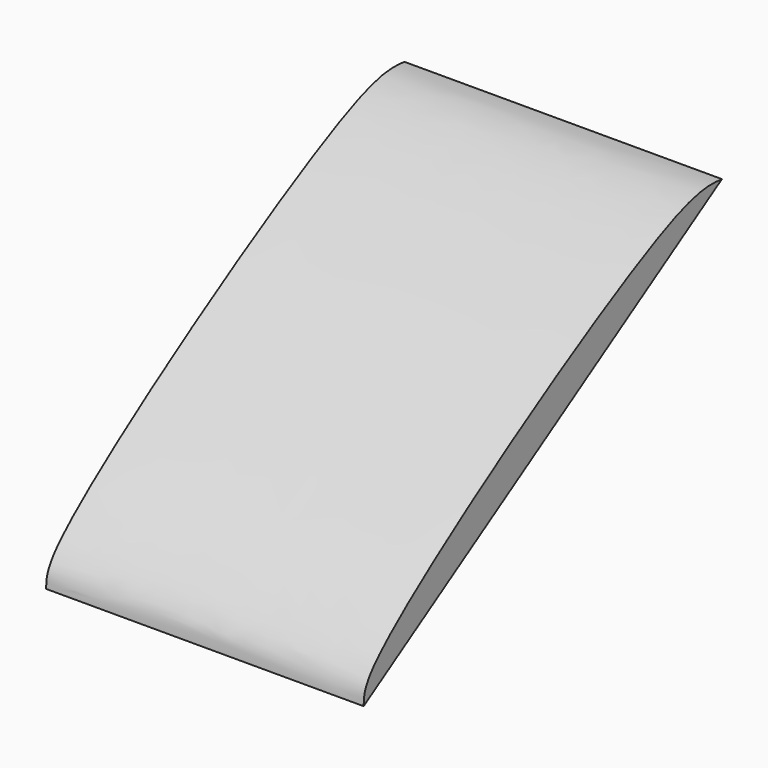
from build123d import *

# Parameters (mm, degrees)
F1_DEPTH  = 457.2
F2_W      = 63.5
F2_H      = 101.6
F3_DEPTH  = 50.8
F5_DEPTH  = 127
F7_DEPTH  = 6.35
F9_DEPTH  = 6.35
F11_DEPTH = 7.62
F12_W     = 19.05
F12_H     = 38.1
F13_DEPTH = 6.35
F14_W     = 9.525
F14_H     = 114.3
F15_DEPTH = 6.35
F17_DEPTH = 19.05
F19_DEPTH = 19.05
F21_DEPTH = 19.05
F23_DEPTH = 127


with BuildPart() as f1:
    # F0 (on Right) → F1 (new body)
    with BuildSketch(Plane.YZ):
        with BuildLine():
            Line((-644.8294241484, -406.0037115008), (0, 0))
            add(Edge.make_bspline(
                [(-644.8294241484, -406.0037115008), (-644.5583562129, -393.7520607079), (-643.3425508393, -338.8004381801), (-93.9791762847, 8.8024420181), (-20.2683336801, 1.8984081269), (0, 0)],
                knots=[0, 0, 0, 0, 0.1722048446, 0.7723804554, 1, 1, 1, 1], degree=3))
        make_face()
    extrude(amount=F1_DEPTH)

    # F2 (on face) → F3 (join)
    with BuildSketch(Plane(origin=(0, 0, 0), x_dir=(1, 0, 0), z_dir=(0, 0.5328132697, -0.8462328401))):
        with Locations((228.6, 381)):
            Rectangle(F2_W, F2_H)
    extrude(amount=F3_DEPTH)

    # F4 (on face) → F5 (cut)
    with BuildSketch(Plane(origin=(196.85, 0, 0), x_dir=(0, -1, 0), z_dir=(-1, 0, 0))):
        with BuildLine():
            Line((287.9840051675, -233.8501769674), (284.600640905, -239.223755502))
            Line((284.600640905, -239.223755502), (306.0949550433, -252.757212552))
            Line((306.0949550433, -252.757212552), (309.4783193058, -247.3836340174))
            Line((309.4783193058, -247.3836340174), (330.9726334441, -260.9170910675))
            ThreePointArc((330.9726334441, -260.9170910675), (317.4401312079, -210.9026606557), (266.4896910292, -220.3167199174))
            Line((266.4896910292, -220.3167199174), (287.9840051675, -233.8501769674))
        make_face()
    extrude(amount=-F5_DEPTH, mode=Mode.SUBTRACT)

    # F6 (on face) → F7 (join)
    with BuildSketch(Plane(origin=(196.85, 0, 0), x_dir=(0, -1, 0), z_dir=(-1, 0, 0))):
        with BuildLine():
            Line((252.3591696976, -218.9235699269), (284.600640905, -239.223755502))
            Line((284.600640905, -239.223755502), (287.9840051675, -233.8501769674))
            Line((287.9840051675, -233.8501769674), (266.4896910292, -220.3167199174))
            ThreePointArc((266.4896910292, -220.3167199174), (317.4401312079, -210.9026606557), (330.9726334441, -260.9170910675))
            Line((330.9726334441, -260.9170910675), (309.4783193058, -247.3836340174))
            Line((309.4783193058, -247.3836340174), (306.0949550433, -252.757212552))
            Line((306.0949550433, -252.757212552), (338.3364262507, -273.057398127))
            Line((338.3364262507, -273.057398127), (365.4033403508, -230.0687698505))
            Line((365.4033403508, -230.0687698505), (279.4260837976, -175.9349416504))
            Line((279.4260837976, -175.9349416504), (252.3591696976, -218.9235699269))
        make_face()
        with BuildLine():
            Line((287.9840051675, -233.8501769674), (284.600640905, -239.223755502))
            Line((284.600640905, -239.223755502), (306.0949550433, -252.757212552))
            Line((306.0949550433, -252.757212552), (309.4783193058, -247.3836340174))
            Line((309.4783193058, -247.3836340174), (330.9726334441, -260.9170910675))
            ThreePointArc((330.9726334441, -260.9170910675), (317.4401312079, -210.9026606557), (266.4896910292, -220.3167199174))
            Line((266.4896910292, -220.3167199174), (287.9840051675, -233.8501769674))
        make_face()
    extrude(amount=F7_DEPTH)

    # F8 (on face) → F9 (join)
    with BuildSketch(Plane.YZ.offset(260.35)):
        with BuildLine():
            Line((-338.3364262507, -273.057398127), (-306.0949550433, -252.757212552))
            Line((-306.0949550433, -252.757212552), (-309.4783193058, -247.3836340174))
            Line((-309.4783193058, -247.3836340174), (-330.9726334441, -260.9170910675))
            ThreePointArc((-330.9726334441, -260.9170910675), (-317.4401312079, -210.9026606557), (-266.4896910292, -220.3167199174))
            Line((-266.4896910292, -220.3167199174), (-287.9840051675, -233.8501769674))
            Line((-287.9840051675, -233.8501769674), (-284.600640905, -239.223755502))
            Line((-284.600640905, -239.223755502), (-252.3591696976, -218.9235699269))
            Line((-252.3591696976, -218.9235699269), (-279.4260837976, -175.9349416504))
            Line((-279.4260837976, -175.9349416504), (-365.4033403508, -230.0687698505))
            Line((-365.4033403508, -230.0687698505), (-338.3364262507, -273.057398127))
        make_face()
        with BuildLine():
            Line((-309.4783193058, -247.3836340174), (-306.0949550433, -252.757212552))
            Line((-306.0949550433, -252.757212552), (-284.600640905, -239.223755502))
            Line((-284.600640905, -239.223755502), (-287.9840051675, -233.8501769674))
            Line((-287.9840051675, -233.8501769674), (-266.4896910292, -220.3167199174))
            ThreePointArc((-266.4896910292, -220.3167199174), (-317.4401312079, -210.9026606557), (-330.9726334441, -260.9170910675))
            Line((-330.9726334441, -260.9170910675), (-309.4783193058, -247.3836340174))
        make_face()
    extrude(amount=F9_DEPTH)

    # F10 (on face) → F11 (cut)
    with BuildSketch(Plane(origin=(0, 27.0669141001, -42.9886282766), x_dir=(1, 0, 0), z_dir=(0, 0.5328132697, -0.8462328401))):
        with BuildLine():
            Line((260.35, 368.3), (196.85, 368.3))
            ThreePointArc((196.85, 368.3), (228.6, 364.3836558631), (260.35, 368.3))
        make_face()
        with BuildLine():
            ThreePointArc((260.35, 393.7), (228.6, 398.6686937584), (196.85, 393.7))
            Line((196.85, 393.7), (260.35, 393.7))
        make_face()
    extrude(amount=-F11_DEPTH, mode=Mode.SUBTRACT)

    # F12 (on face) → F13 (join)
    with BuildSketch(Plane(origin=(0, 0, 0), x_dir=(1, 0, 0), z_dir=(0, 0.5328132697, -0.8462328401))):
        with Locations((276.225, 304.8)):
            Rectangle(F12_W, F12_H)
        with Locations((180.975, 304.8)):
            Rectangle(F12_W, F12_H)
        with Locations((180.975, 457.2)):
            Rectangle(F12_W, F12_H)
        with Locations((276.225, 457.2)):
            Rectangle(F12_W, F12_H)
    extrude(amount=F13_DEPTH)

    # F14 (on face) → F15 (join)
    with BuildSketch(Plane(origin=(0, 0, 0), x_dir=(1, 0, 0), z_dir=(0, 0.5328132697, -0.8462328401))):
        with Locations((280.9875, 381)):
            Rectangle(F14_W, F14_H)
        with Locations((176.2125, 381)):
            Rectangle(F14_W, F14_H)
    extrude(amount=F15_DEPTH)

    # F16 (on face) → F17 (join, through all)
    with BuildSketch(Plane(origin=(171.45, 0, 0), x_dir=(0, -1, 0), z_dir=(-1, 0, 0))):
        with BuildLine():
            ThreePointArc((367.3831611706, -238.8191686221), (288.3689781086, -256.7769374998), (270.4112092309, -177.7627544378))
            Line((270.4112092309, -177.7627544378), (238.4276697931, -157.6249703474))
            ThreePointArc((238.4276697931, -157.6249703474), (268.2808838741, -288.9791123035), (399.6350258302, -259.1258982226))
            Line((399.6350258302, -259.1258982226), (367.3831611706, -238.8191686221))
        make_face()
        with BuildLine():
            ThreePointArc((239.1093056989, -187.7121895128), (248.2100145695, -184.8899649175), (249.5985309983, -194.3165165532))
            ThreePointArc((249.5985309983, -194.3165165532), (281.2555246608, -268.0747753287), (361.4511619568, -264.7422471567))
            ThreePointArc((361.4511619568, -264.7422471567), (370.7846763643, -261.84782714), (372.2087124782, -271.5155197072))
            ThreePointArc((372.2087124782, -271.5155197072), (373.6678203851, -278.069248149), (367.3998277743, -275.6624617016))
            ThreePointArc((367.3998277743, -275.6624617016), (359.600539495, -281.1588159356), (351.2112735384, -285.7040358686))
            ThreePointArc((351.2112735384, -285.7040358686), (350.5826225392, -292.3887310968), (345.3595430971, -288.1697509458))
            ThreePointArc((345.3595430971, -288.1697509458), (336.2472580827, -290.999074071), (326.8663458105, -292.7418570382))
            ThreePointArc((326.8663458105, -292.7418570382), (324.2109582174, -298.908644622), (320.5397892842, -293.2870015315))
            ThreePointArc((320.5397892842, -293.2870015315), (310.9990248614, -293.1746549338), (301.5370588891, -291.9458313221))
            ThreePointArc((301.5370588891, -291.9458313221), (297.1126896264, -296.9961094334), (295.3497866634, -290.5174887842))
            ThreePointArc((295.3497866634, -290.5174887842), (286.3066520823, -287.4743777976), (277.6820927997, -283.3932278725))
            ThreePointArc((277.6820927997, -283.3932278725), (271.9182094781, -286.8367727653), (272.2346951196, -280.1300456044))
            ThreePointArc((272.2346951196, -280.1300456044), (264.5669953666, -274.4515609449), (257.6170172155, -267.9142364747))
            ThreePointArc((257.6170172155, -267.9142364747), (251.0731122849, -269.416787849), (253.4382656928, -263.1329672174))
            ThreePointArc((253.4382656928, -263.1329672174), (247.8902941341, -255.370311801), (243.2895222041, -247.011382134))
            ThreePointArc((243.2895222041, -247.011382134), (236.6008037693, -246.4270893363), (240.7850426635, -241.1761373036))
            ThreePointArc((240.7850426635, -241.1761373036), (237.8953334828, -232.0828217157), (236.0903585556, -222.713676982))
            ThreePointArc((236.0903585556, -222.713676982), (229.9060915749, -220.0992565331), (235.5032574787, -216.3908759946))
            ThreePointArc((235.5032574787, -216.3908759946), (235.6875620889, -205.0479961951), (237.4482217292, -193.8410801176))
            ThreePointArc((237.4482217292, -193.8410801176), (232.5687062994, -189.2290652061), (239.1093056989, -187.7121895128))
        make_face(mode=Mode.SUBTRACT)
    extrude(amount=-F17_DEPTH)

    # F18 (on face) → F19 (join)
    with BuildSketch(Plane.YZ.offset(285.75)):
        with BuildLine():
            ThreePointArc((-270.5689041654, -177.9978801358), (-288.5149065441, -257.0147364807), (-367.5317628891, -239.068734102))
            Line((-367.5317628891, -239.068734102), (-399.5123031789, -259.2112807586))
            ThreePointArc((-399.5123031789, -259.2112807586), (-268.1537171245, -289.044934068), (-238.320063815, -157.6863480136))
            Line((-238.320063815, -157.6863480136), (-270.5689041654, -177.9978801358))
        make_face()
        with BuildLine():
            ThreePointArc((-372.0841451457, -271.5968179501), (-370.6970324756, -262.1700596497), (-361.5959034378, -264.9909289928))
            ThreePointArc((-361.5959034378, -264.9909289928), (-281.3997707716, -268.3115148932), (-249.7537610805, -194.5485427732))
            ThreePointArc((-249.7537610805, -194.5485427732), (-248.331164635, -184.8806382546), (-238.997219312, -187.7736683504))
            ThreePointArc((-238.997219312, -187.7736683504), (-232.4563941014, -189.2895700416), (-237.3352226845, -193.902311529))
            ThreePointArc((-237.3352226845, -193.902311529), (-235.7483929759, -203.310859717), (-235.2742480634, -212.8404973875))
            ThreePointArc((-235.2742480634, -212.8404973875), (-229.5174036152, -216.2957968495), (-235.5790353354, -219.1831785807))
            ThreePointArc((-235.5790353354, -219.1831785807), (-236.9647482072, -228.6234437977), (-239.4464083444, -237.8364872955))
            ThreePointArc((-239.4464083444, -237.8364872955), (-235.0323538545, -242.895783228), (-241.6883942228, -243.7775309177))
            ThreePointArc((-241.6883942228, -243.7775309177), (-245.9121403787, -252.3331592372), (-251.1087141332, -260.3353107443))
            ThreePointArc((-251.1087141332, -260.3353107443), (-248.4659159709, -266.5075040536), (-255.0702720454, -265.2980276321))
            ThreePointArc((-255.0702720454, -265.2980276321), (-261.7220580916, -272.1385356487), (-269.1291209948, -278.1530370143))
            ThreePointArc((-269.1291209948, -278.1530370143), (-268.5141120454, -284.8390011456), (-274.4257078095, -281.6557028726))
            ThreePointArc((-274.4257078095, -281.6557028726), (-282.8598537654, -286.1170916164), (-291.7584121219, -289.560123232))
            ThreePointArc((-291.7584121219, -289.560123232), (-293.230890482, -296.1108605838), (-297.8758952364, -291.2627389678))
            ThreePointArc((-297.8758952364, -291.2627389678), (-307.2737098275, -292.9119473966), (-316.7999924715, -293.4492987853))
            ThreePointArc((-316.7999924715, -293.4492987853), (-320.2170266349, -299.2289380388), (-323.1445559768, -293.1865937648))
            ThreePointArc((-323.1445559768, -293.1865937648), (-332.5938059019, -291.8635354209), (-341.8231093104, -289.4430466017))
            ThreePointArc((-341.8231093104, -289.4430466017), (-346.8530123381, -293.8905658996), (-347.7788949072, -287.24052125))
            ThreePointArc((-347.7788949072, -287.24052125), (-357.928637458, -282.1732126459), (-367.2746429584, -275.7430437893))
            ThreePointArc((-367.2746429584, -275.7430437893), (-373.542277096, -278.1507636005), (-372.0841451457, -271.5968179501))
        make_face(mode=Mode.SUBTRACT)
    extrude(amount=-F19_DEPTH)

    # F20 (on face) → F21 (join)
    with BuildSketch(Plane.YZ.offset(285.75)):
        with BuildLine():
            ThreePointArc((-237.3352226845, -193.902311529), (-232.4563941014, -189.2895700416), (-238.997219312, -187.7736683504))
            Line((-238.997219312, -187.7736683504), (-237.3352226845, -193.902311529))
        make_face()
        with BuildLine():
            ThreePointArc((-235.5790353354, -219.1831785807), (-229.5174036152, -216.2957968495), (-235.2742480634, -212.8404973875))
            Line((-235.2742480634, -212.8404973875), (-235.5790353354, -219.1831785807))
        make_face()
        with BuildLine():
            ThreePointArc((-241.6883942228, -243.7775309177), (-235.0323538545, -242.895783228), (-239.4464083444, -237.8364872955))
            Line((-239.4464083444, -237.8364872955), (-241.6883942228, -243.7775309177))
        make_face()
        with BuildLine():
            ThreePointArc((-255.0702720454, -265.2980276321), (-248.4659159709, -266.5075040536), (-251.1087141332, -260.3353107443))
            Line((-251.1087141332, -260.3353107443), (-255.0702720454, -265.2980276321))
        make_face()
        with BuildLine():
            ThreePointArc((-274.4257078095, -281.6557028726), (-268.5141120454, -284.8390011456), (-269.1291209948, -278.1530370143))
            Line((-269.1291209948, -278.1530370143), (-274.4257078095, -281.6557028726))
        make_face()
        with BuildLine():
            Line((-291.7584121219, -289.560123232), (-297.8758952364, -291.2627389678))
            ThreePointArc((-297.8758952364, -291.2627389678), (-293.230890482, -296.1108605838), (-291.7584121219, -289.560123232))
        make_face()
        with BuildLine():
            Line((-316.7999924715, -293.4492987853), (-323.1445559768, -293.1865937648))
            ThreePointArc((-323.1445559768, -293.1865937648), (-320.2170266349, -299.2289380388), (-316.7999924715, -293.4492987853))
        make_face()
        with BuildLine():
            Line((-341.8231093104, -289.4430466017), (-347.7788949072, -287.24052125))
            ThreePointArc((-347.7788949072, -287.24052125), (-346.8530123381, -293.8905658996), (-341.8231093104, -289.4430466017))
        make_face()
    extrude(amount=-F21_DEPTH)

    # F22 (on face) → F23 (cut)
    with BuildSketch(Plane(origin=(171.45, 0, 0), x_dir=(0, -1, 0), z_dir=(-1, 0, 0))):
        with BuildLine():
            ThreePointArc((345.3595430971, -288.1697509458), (350.5826225392, -292.3887310968), (351.2112735384, -285.7040358686))
            Line((351.2112735384, -285.7040358686), (345.3595430971, -288.1697509458))
        make_face()
        with BuildLine():
            ThreePointArc((320.5397892842, -293.2870015315), (324.2109582174, -298.908644622), (326.8663458105, -292.7418570382))
            Line((326.8663458105, -292.7418570382), (320.5397892842, -293.2870015315))
        make_face()
        with BuildLine():
            ThreePointArc((295.3497866634, -290.5174887842), (297.1126896264, -296.9961094334), (301.5370588891, -291.9458313221))
            Line((301.5370588891, -291.9458313221), (295.3497866634, -290.5174887842))
        make_face()
        with BuildLine():
            ThreePointArc((272.2346951196, -280.1300456044), (271.9182094781, -286.8367727653), (277.6820927997, -283.3932278725))
            Line((277.6820927997, -283.3932278725), (272.2346951196, -280.1300456044))
        make_face()
        with BuildLine():
            ThreePointArc((253.4382656928, -263.1329672174), (251.0731122849, -269.416787849), (257.6170172155, -267.9142364747))
            Line((257.6170172155, -267.9142364747), (253.4382656928, -263.1329672174))
        make_face()
        with BuildLine():
            Line((243.2895222041, -247.011382134), (240.7850426635, -241.1761373036))
            ThreePointArc((240.7850426635, -241.1761373036), (236.6008037693, -246.4270893363), (243.2895222041, -247.011382134))
        make_face()
        with BuildLine():
            Line((236.0903585556, -222.713676982), (235.5032574787, -216.3908759946))
            ThreePointArc((235.5032574787, -216.3908759946), (229.9060915749, -220.0992565331), (236.0903585556, -222.713676982))
        make_face()
        with BuildLine():
            Line((237.4482217292, -193.8410801176), (239.1093056989, -187.7121895128))
            ThreePointArc((239.1093056989, -187.7121895128), (232.5687062994, -189.2290652061), (237.4482217292, -193.8410801176))
        make_face()
    extrude(amount=-F23_DEPTH, mode=Mode.SUBTRACT)


solid = f1.part
